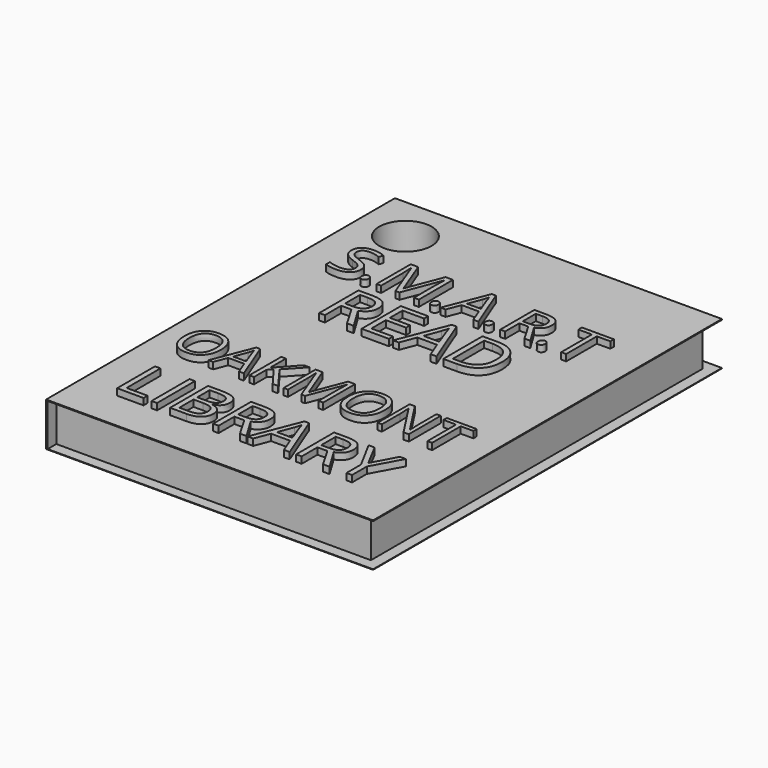
from build123d import *

# Parameters (mm, degrees)
F0_W           = 38.1
F0_H           = 50.8
F1_DEPTH       = 5.08
F2_TEXT_SIZE   = 6.9656132833
F2_TEXT_SIZE_2 = 8.0004921563
F2_TEXT_SIZE_3 = 6.5134227154
F2_TEXT_SIZE_4 = 7.7366542397
F3_DEPTH       = 0.762
F5_DEPTH       = 1.27
F6_W           = 49.53
F6_H           = 4.9295544522
F7_DEPTH       = 1.27
F8_W           = 36.6466352386
F8_H           = 4.9295544522
F9_DEPTH       = 1.27
F10_R          = 3.048
F11_DEPTH      = 127


# Not quite as in the source:
# - Text() gives the source's letters only with a copy of the font that has no kerning and outlines rounded to 1/6400 em; it was checked with that copy


with BuildPart() as f1:
    # F0 (on Top) → F1 (new body)
    with BuildSketch(Plane.XY):
        with Locations((-32.2314618772, 11.2663237378)):
            Rectangle(F0_W, F0_H)
    extrude(amount=F1_DEPTH)

    # F2 (on face) → F3 (join)
    with BuildSketch(Plane.XY.offset(5.08)):
        with Locations((-47.4714618772, 21.2832182722)):
            Text('S.M.A.R.T', F2_TEXT_SIZE, font='Open Sans', text_align=(TextAlign.LEFT, TextAlign.BOTTOM))
        with Locations((-42.3914618772, 13.5443307473)):
            Text('READ', F2_TEXT_SIZE_2, font='Open Sans', text_align=(TextAlign.LEFT, TextAlign.BOTTOM))
        with Locations((-48.7414618772, 0)):
            Text('OAKMONT', F2_TEXT_SIZE_3, font='Open Sans', text_align=(TextAlign.LEFT, TextAlign.BOTTOM))
        with Locations((-47.4714618772, -9.5037243787)):
            Text('LIBRARY', F2_TEXT_SIZE_4, font='Open Sans', text_align=(TextAlign.LEFT, TextAlign.BOTTOM))
    extrude(amount=F3_DEPTH)

    # F4 (on face) → F5 (cut)
    with BuildSketch(Plane(origin=(0, 36.6663237378, 0), x_dir=(-1, 0, 0), z_dir=(0, 1, 0))):
        Polygon((51.1291287839, 0.0574870137), (51.1291287839, 4.9870414659), (13.2959568873, 4.9870414659), (13.1814618772, 4.9870414659), (13.1814618772, 0.0574870137), (13.2959568873, 0.0574870137), align=None)
    extrude(amount=-F5_DEPTH, mode=Mode.SUBTRACT)

    # F6 (on face) → F7 (cut)
    with BuildSketch(Plane.YZ.offset(-13.1814618772)):
        with Locations((10.6313237378, 2.5222642398)):
            Rectangle(F6_W, F6_H)
    extrude(amount=-F7_DEPTH, mode=Mode.SUBTRACT)

    # F8 (on face) → F9 (cut)
    with BuildSketch(Plane.XZ.offset(14.1336762622)):
        with Locations((-32.7747794965, 2.5222642398)):
            Rectangle(F8_W, F8_H)
    extrude(amount=-F9_DEPTH, mode=Mode.SUBTRACT)

    # F10 (on face) → F11 (cut)
    with BuildSketch(Plane.XY.offset(5.08)):
        with Locations((-45.8433750901, 31.4015158541)):
            Circle(F10_R)
    extrude(amount=-F11_DEPTH, mode=Mode.SUBTRACT)


solid = f1.part
